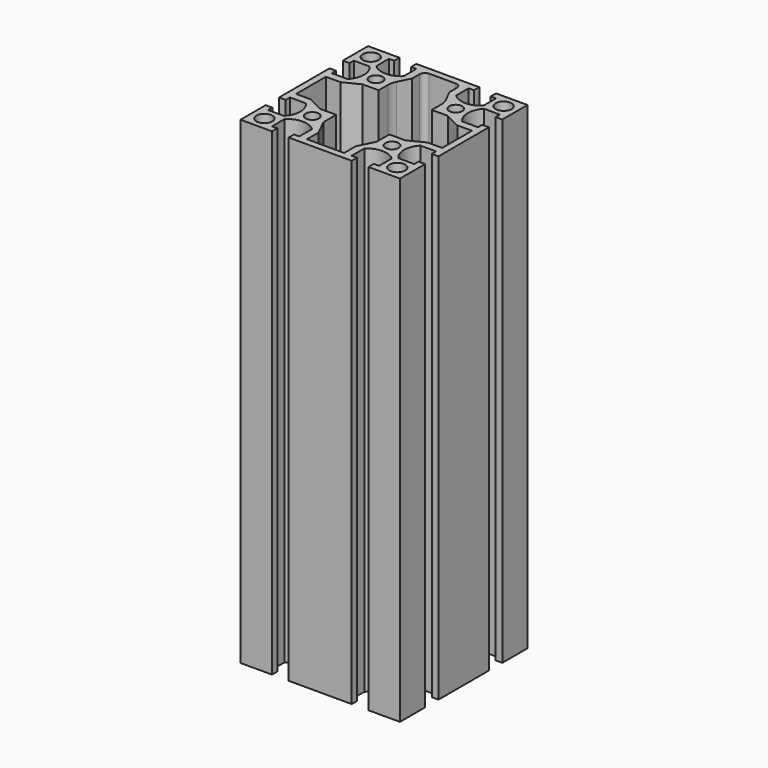
from build123d import *

# Parameters (mm, degrees)
F0_R     = 3
F0_R_2   = 2.5
F1_DEPTH = 180
F2_R     = 2
F3_R     = 7


# Not quite as in the source:
# - a feature names something its author has since deleted; it is built from what else it names


with BuildPart() as f1:
    # F0 (on Top) → F1 (new body)
    with BuildSketch(Plane.XY):
        with BuildLine():
            Line((18.15, -30), (30, -30))
            Line((30, -30), (30, -18.15))
            Line((30, -18.15), (27.5, -18.15))
            Line((27.5, -18.15), (27.5, -20.15))
            Line((27.5, -20.15), (21.5477069044, -20.15))
            ThreePointArc((21.5477069044, -20.15), (19.5, -15), (21.5477069044, -9.85))
            Line((21.5477069044, -9.85), (27.5, -9.85))
            Line((27.5, -9.85), (27.5, -11.85))
            Line((27.5, -11.85), (30, -11.85))
            Line((30, -11.85), (30, 11.85))
            Line((30, 11.85), (27.5, 11.85))
            Line((27.5, 11.85), (27.5, 9.85))
            Line((27.5, 9.85), (21.5477069044, 9.85))
            ThreePointArc((21.5477069044, 9.85), (19.5, 15), (21.5477069044, 20.15))
            Line((21.5477069044, 20.15), (27.5, 20.15))
            Line((27.5, 20.15), (27.5, 18.15))
            Line((27.5, 18.15), (30, 18.15))
            Line((30, 18.15), (30, 30))
            Line((30, 30), (18.15, 30))
            Line((18.15, 30), (18.15, 27.5))
            Line((18.15, 27.5), (20.15, 27.5))
            Line((20.15, 27.5), (20.15, 21.5477069044))
            ThreePointArc((20.15, 21.5477069044), (15, 19.5), (9.85, 21.5477069044))
            Line((9.85, 21.5477069044), (9.85, 27.5))
            Line((9.85, 27.5), (11.85, 27.5))
            Line((11.85, 27.5), (11.85, 30))
            Line((11.85, 30), (-11.85, 30))
            Line((-11.85, 30), (-11.85, 27.5))
            Line((-11.85, 27.5), (-9.85, 27.5))
            Line((-9.85, 27.5), (-9.85, 21.5477069044))
            ThreePointArc((-9.85, 21.5477069044), (-15, 19.5), (-20.15, 21.5477069044))
            Line((-20.15, 21.5477069044), (-20.15, 27.5))
            Line((-20.15, 27.5), (-18.15, 27.5))
            Line((-18.15, 27.5), (-18.15, 30))
            Line((-18.15, 30), (-30, 30))
            Line((-30, 30), (-30, 18.15))
            Line((-30, 18.15), (-27.5, 18.15))
            Line((-27.5, 18.15), (-27.5, 20.15))
            Line((-27.5, 20.15), (-21.5477069044, 20.15))
            ThreePointArc((-21.5477069044, 20.15), (-19.5, 15), (-21.5477069044, 9.85))
            Line((-21.5477069044, 9.85), (-27.5, 9.85))
            Line((-27.5, 9.85), (-27.5, 11.85))
            Line((-27.5, 11.85), (-30, 11.85))
            Line((-30, 11.85), (-30, -11.85))
            Line((-30, -11.85), (-27.5, -11.85))
            Line((-27.5, -11.85), (-27.5, -9.85))
            Line((-27.5, -9.85), (-21.5477069044, -9.85))
            ThreePointArc((-21.5477069044, -9.85), (-19.5, -15), (-21.5477069044, -20.15))
            Line((-21.5477069044, -20.15), (-27.5, -20.15))
            Line((-27.5, -20.15), (-27.5, -18.15))
            Line((-27.5, -18.15), (-30, -18.15))
            Line((-30, -18.15), (-30, -30))
            Line((-30, -30), (-18.15, -30))
            Line((-18.15, -30), (-18.15, -27.5))
            Line((-18.15, -27.5), (-20.15, -27.5))
            Line((-20.15, -27.5), (-20.15, -21.5477069044))
            ThreePointArc((-20.15, -21.5477069044), (-15, -19.5), (-9.85, -21.5477069044))
            Line((-9.85, -21.5477069044), (-9.85, -27.5))
            Line((-9.85, -27.5), (-11.85, -27.5))
            Line((-11.85, -27.5), (-11.85, -30))
            Line((-11.85, -30), (11.85, -30))
            Line((11.85, -30), (11.85, -27.5))
            Line((11.85, -27.5), (9.85, -27.5))
            Line((9.85, -27.5), (9.85, -21.5477069044))
            ThreePointArc((9.85, -21.5477069044), (15, -19.5), (20.15, -21.5477069044))
            Line((20.15, -21.5477069044), (20.15, -27.5))
            Line((20.15, -27.5), (18.15, -27.5))
            Line((18.15, -27.5), (18.15, -30))
        make_face()
        with Locations((-25, -25)):
            Circle(F0_R, mode=Mode.SUBTRACT)
        with Locations((-15, -15)):
            Circle(F0_R_2, mode=Mode.SUBTRACT)
        with Locations((25, -25)):
            Circle(F0_R, mode=Mode.SUBTRACT)
        with Locations((15, -15)):
            Circle(F0_R_2, mode=Mode.SUBTRACT)
        with Locations((-25, 25)):
            Circle(F0_R, mode=Mode.SUBTRACT)
        with Locations((-15, 15)):
            Circle(F0_R_2, mode=Mode.SUBTRACT)
        Polygon((-7, 22), (-7, 27.5), (0, 27.5), (7, 27.5), (7, 22), (10, 16), (10, 10), (16, 10), (22, 7), (27.5, 7), (27.5, 0), (27.5, -7), (22, -7), (16, -10), (10, -10), (10, -16), (7, -22), (7, -27.5), (0, -27.5), (-7, -27.5), (-7, -22), (-10, -16), (-10, -10), (-16, -10), (-22, -7), (-27.5, -7), (-27.5, 0), (-27.5, 7), (-22, 7), (-16, 10), (-10, 10), (-10, 16), align=None, mode=Mode.SUBTRACT)
        with Locations((15, 15)):
            Circle(F0_R_2, mode=Mode.SUBTRACT)
        with Locations((25, 25)):
            Circle(F0_R, mode=Mode.SUBTRACT)
    extrude(amount=F1_DEPTH)

    # F2
    f2_edges = [f1.edges().sort_by_distance(p)[0] for p in [
        (-7, 27.5, 90),
        (7, 27.5, 90),
    ]]
    fillet(f2_edges, radius=F2_R)

    # F3
    f3_edges = [f1.edges().sort_by_distance(p)[0] for p in [
        (-10, 16, 90),
        (10, 16, 90),
    ]]
    fillet(f3_edges, radius=F3_R)


solid = f1.part
